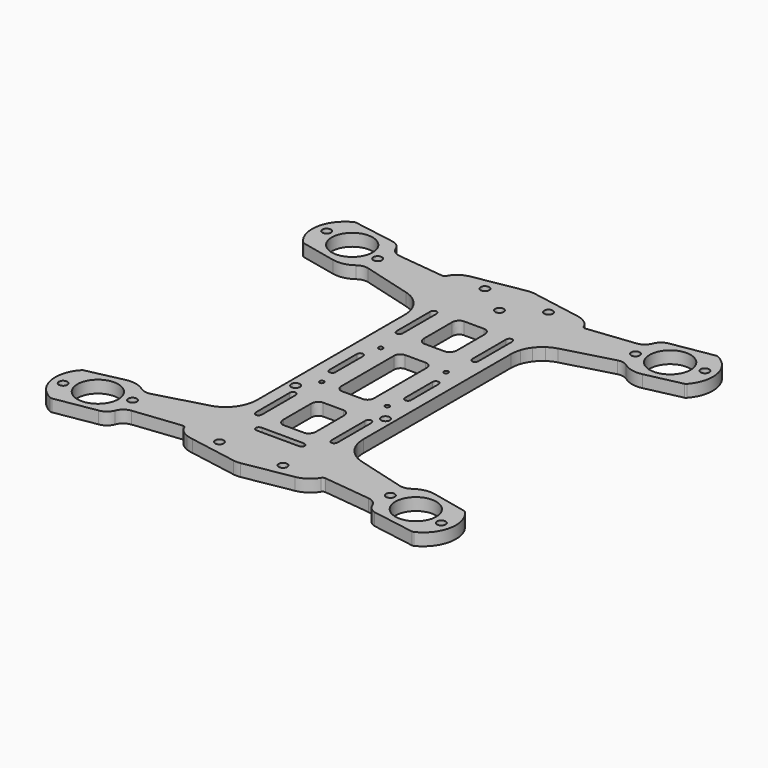
from build123d import *

# Parameters (mm, degrees)
F0_R     = 1.05
F0_R_2   = 5
F0_R_3   = 0.55
F1_DEPTH = 3


# Not quite as in the source:
# - ends of sketch curves that miss each other by under 0.0002 mm in the source are joined


with BuildPart() as f1:
    # F0 (on Top) → F1 (new body)
    with BuildSketch(Plane.XY):
        with BuildLine():
            Line((12.547114, 42.881202), (0.85655, 44.92619))
            ThreePointArc((0.85655, 44.92619), (-0.005, 45.000977), (-0.8665501465, 44.9261908375))
            Line((-0.8665501465, 44.9261908375), (-12.557114, 42.881202))
            ThreePointArc((-12.557114, 42.881202), (-13.3811659144, 42.726197173), (-14.1806832522, 42.4734916576))
            ThreePointArc((-14.1806832522, 42.4734916576), (-14.8442493228, 42.1649785483), (-15.4590972968, 41.7681633969))
            ThreePointArc((-15.4590972968, 41.7681633969), (-15.9947726207, 41.2927995203), (-16.4437235489, 40.7348013706))
            ThreePointArc((-16.4437235489, 40.7348013706), (-16.6010065857, 40.474068763), (-16.7309251323, 40.1986770543))
            ThreePointArc((-16.7309251323, 40.1986770543), (-17.0633376993, 39.8142902587), (-17.5602140107, 39.7076819051))
            Line((-17.5602140107, 39.7076819051), (-28.976888, 40.990102))
            ThreePointArc((-28.976888, 40.990102), (-30.4889144129, 41.6072597908), (-31.4536189137, 42.9250050321))
            ThreePointArc((-31.4536189137, 42.9250050321), (-32.2669695523, 44.1162796633), (-33.5422899426, 44.790247231))
            Line((-33.5422899426, 44.790247231), (-44.024355, 46.547073))
            ThreePointArc((-44.024355, 46.547073), (-44.2703960354, 46.5499421734), (-44.5056712286, 46.4779004714))
            ThreePointArc((-44.5056712286, 46.4779004714), (-48.8678182924, 40.8066015152), (-46.9486082896, 33.9139537381))
            ThreePointArc((-46.9486082896, 33.9139537381), (-46.756758402, 33.7585868692), (-46.5266729937, 33.6691110288))
            Line((-46.5266729937, 33.6691110288), (-37.857414, 31.767143))
            ThreePointArc((-37.857414, 31.767143), (-35.3359003634, 31.7563904573), (-33.0326374155, 32.7826095689))
            ThreePointArc((-33.0326374155, 32.7826095689), (-31.8035160934, 33.3109660693), (-30.4669251472, 33.2524484654))
            Line((-30.4669251472, 33.2524484654), (-18.56562, 29.976315))
            ThreePointArc((-18.56562, 29.976315), (-17.4138061916, 29.5556879599), (-16.3477285533, 28.9498161915))
            ThreePointArc((-16.3477285533, 28.9498161915), (-15.3811482934, 28.1647172936), (-14.555782994, 27.2322850045))
            ThreePointArc((-14.555782994, 27.2322850045), (-13.8911084628, 26.1763608601), (-13.404806368, 25.0273272092))
            ThreePointArc((-13.404806368, 25.0273272092), (-13.1055926689, 23.8032308073), (-13.005, 22.547117))
            Line((-13.005, 22.547117), (-13.005, -22.545163))
            ThreePointArc((-13.005, -22.545163), (-13.1056391598, -23.8016289395), (-13.4049904879, -25.0260568385))
            ThreePointArc((-13.4049904879, -25.0260568385), (-13.8915403308, -26.1754629051), (-14.5565378338, -27.2317031244))
            ThreePointArc((-14.5565378338, -27.2317031244), (-15.3822911127, -28.1644003108), (-16.3492958707, -28.949699189))
            ThreePointArc((-16.3492958707, -28.949699189), (-17.4159327082, -29.5557766888), (-18.5683238155, -29.976536675))
            Line((-18.5683238155, -29.976536675), (-30.468827, -33.252449))
            ThreePointArc((-30.468827, -33.252449), (-31.8054180934, -33.3109660693), (-33.0345392685, -32.7826093676))
            ThreePointArc((-33.0345392685, -32.7826093676), (-35.3378023634, -31.7563904573), (-37.8593158453, -31.7671437053))
            Line((-37.8593158453, -31.7671437053), (-46.528575, -33.669111))
            ThreePointArc((-46.528575, -33.669111), (-46.758660402, -33.7585868692), (-46.9505100734, -33.9139539336))
            ThreePointArc((-46.9505100734, -33.9139539336), (-48.8697202924, -40.8066015152), (-44.5075733347, -46.4779006903))
            ThreePointArc((-44.5075733347, -46.4779006903), (-44.2722980354, -46.5499421734), (-44.0262569999, -46.5470730008))
            Line((-44.0262569999, -46.5470730008), (-34.00125, -44.866851))
            ThreePointArc((-34.00125, -44.866851), (-32.4476725244, -44.2639383706), (-31.4555210863, -42.9250049679))
            ThreePointArc((-31.4555210863, -42.9250049679), (-30.4908164129, -41.6072597908), (-28.9787899602, -40.9901023543))
            Line((-28.9787899602, -40.9901023543), (-17.559317, -39.707367))
            ThreePointArc((-17.559317, -39.707367), (-17.0624979522, -39.8139429564), (-16.7300789977, -40.1982409991))
            ThreePointArc((-16.7300789977, -40.1982409991), (-16.6002219721, -40.4733867622), (-16.4430270568, -40.7338820384))
            ThreePointArc((-16.4430270568, -40.7338820384), (-15.9941324256, -41.2916401808), (-15.4585510869, -41.7667751162))
            ThreePointArc((-15.4585510869, -41.7667751162), (-14.8438267074, -42.1633861463), (-14.1804188227, -42.4717305375))
            ThreePointArc((-14.1804188227, -42.4717305375), (-13.3810245241, -42.7243184881), (-12.557113935, -42.8792484861))
            Line((-12.557113935, -42.8792484861), (-0.86655, -44.924237))
            ThreePointArc((-0.86655, -44.924237), (-0.005, -44.999023), (0.8565499768, -44.9242368672))
            Line((0.8565499768, -44.9242368672), (12.547114, -42.879249))
            ThreePointArc((12.547114, -42.879249), (14.9016711671, -41.9206209342), (16.6479221608, -40.0730510972))
            ThreePointArc((16.6479221608, -40.0730510972), (16.9791102944, -39.7692325356), (17.4218459122, -39.6919257817))
            Line((17.4218459122, -39.6919257817), (28.97879, -40.990102))
            ThreePointArc((28.97879, -40.990102), (30.4908164129, -41.6072597908), (31.4555209137, -42.9250050321))
            ThreePointArc((31.4555209137, -42.9250050321), (32.2688715523, -44.1162796633), (33.5441919426, -44.790247231))
            Line((33.5441919426, -44.790247231), (44.026257, -46.547073))
            ThreePointArc((44.026257, -46.547073), (44.2722980354, -46.5499421734), (44.5075732286, -46.4779004714))
            ThreePointArc((44.5075732286, -46.4779004714), (48.8697202924, -40.8066015152), (46.9505102896, -33.9139537381))
            ThreePointArc((46.9505102896, -33.9139537381), (46.758660402, -33.7585868692), (46.5285749937, -33.6691110288))
            Line((46.5285749937, -33.6691110288), (37.859316, -31.767143))
            ThreePointArc((37.859316, -31.767143), (35.3378023634, -31.7563904573), (33.0345394155, -32.7826095689))
            ThreePointArc((33.0345394155, -32.7826095689), (31.8054180934, -33.3109660693), (30.4688271472, -33.2524484654))
            Line((30.4688271472, -33.2524484654), (18.559028, -29.973977))
            ThreePointArc((18.559028, -29.973977), (17.4064503868, -29.5533376341), (16.3395788739, -28.9474021844))
            ThreePointArc((16.3395788739, -28.9474021844), (15.3725598378, -28.1624472168), (14.5467336983, -27.2300892259))
            ThreePointArc((14.5467336983, -27.2300892259), (13.8816539165, -26.1741955031), (13.3950152055, -25.0250979319))
            ThreePointArc((13.3950152055, -25.0250979319), (13.0956458116, -23.8011576138), (12.995, -22.545163))
            Line((12.995, -22.545163), (12.995, 22.547117))
            ThreePointArc((12.995, 22.547117), (13.0955831803, 23.8028717729), (13.3947679478, 25.0266060173))
            ThreePointArc((13.3947679478, 25.0266060173), (13.8810491707, 26.1753648065), (14.5456781251, 27.2310089064))
            ThreePointArc((14.5456781251, 27.2310089064), (15.3709730893, 28.1631793406), (16.3374399089, 28.9480331332))
            ThreePointArc((16.3374399089, 28.9480331332), (17.4034883055, 29.5537691736), (18.5552417544, 29.9742918988))
            Line((18.5552417544, 29.9742918988), (30.463818, 33.252426))
            ThreePointArc((30.463818, 33.252426), (31.800408437, 33.3109440064), (33.0295292685, 32.7825873676))
            ThreePointArc((33.0295292685, 32.7825873676), (35.3327921796, 31.756367496), (37.8543060546, 31.7671207512))
            Line((37.8543060546, 31.7671207512), (46.523565, 33.669089))
            ThreePointArc((46.523565, 33.669089), (46.7536509796, 33.7585646241), (46.9455010734, 33.9139319336))
            ThreePointArc((46.9455010734, 33.9139319336), (48.8647103142, 40.8065794027), (44.5025641443, 46.4778782976))
            ThreePointArc((44.5025641443, 46.4778782976), (44.2672890354, 46.5499201734), (44.0212479999, 46.5470510008))
            Line((44.0212479999, 46.5470510008), (33.99624, 44.866829))
            ThreePointArc((33.99624, 44.866829), (32.4426631637, 44.2639150954), (31.4505120863, 42.9249819679))
            ThreePointArc((31.4505120863, 42.9249819679), (30.4858074569, 41.6072368251), (28.9737810711, 40.9900793668))
            Line((28.9737810711, 40.9900793668), (17.550624, 39.706931))
            ThreePointArc((17.550624, 39.706931), (17.0537216639, 39.8135552662), (16.7213123855, 40.1979831583))
            ThreePointArc((16.7213123855, 40.1979831583), (16.5913653828, 40.4734865873), (16.434041461, 40.7343266362))
            ThreePointArc((16.434041461, 40.7343266362), (15.9850652254, 41.2924356233), (15.4493465609, 41.76790475))
            ThreePointArc((15.4493465609, 41.76790475), (14.8344418499, 42.164812335), (14.1708039539, 42.4734028797))
            ThreePointArc((14.1708039539, 42.4734028797), (13.371230664, 42.7261632475), (12.547114, 42.881202))
        make_face()
        with Locations((-46.26, -40.3)):
            Circle(F0_R, mode=Mode.SUBTRACT)
        with Locations((-38.895613, -38.887486)):
            Circle(F0_R_2, mode=Mode.SUBTRACT)
        with Locations((-31.53, -37.48)):
            Circle(F0_R, mode=Mode.SUBTRACT)
        with Locations((-7.783131, -40.597392)):
            Circle(F0_R, mode=Mode.SUBTRACT)
        with BuildLine():
            add(Edge.make_bspline(
                [(5.0933147946, -32.4777851358), (5.9933122632, -32.4797918895), (5.9949847622, -31.7297939995), (5.9966572612, -30.9797961094), (5.0966597937, -30.9777888655)],
                knots=[4.7123893072, 4.7123893072, 4.7123893072, 6.2831853072, 6.2831853072, 7.8539813072, 7.8539813072, 7.8539813072], degree=2, weights=[1, 0.7071068967, 1, 0.7071068967, 1]))
            Line((5.0933147946, -32.4777851358), (-5.10666, -32.455041))
            add(Edge.make_bspline(
                [(-5.1033142063, -30.9550448655), (-6.0033121239, -30.9530376206), (-6.0049847619, -31.7030358853), (-6.0066574, -32.4530341501), (-5.10666, -32.455041)],
                knots=[1.570796, 1.570796, 1.570796, 3.1415925, 3.1415925, 4.712389, 4.712389, 4.712389], degree=2, weights=[1, 0.7071067199, 1, 0.7071067199, 1]))
            Line((-5.1033142063, -30.9550448655), (5.0966597937, -30.9777888655))
        make_face(mode=Mode.SUBTRACT)
        with BuildLine():
            add(Edge.make_bspline(
                [(-8.505, -16.4296902941), (-8.5049997549, -15.5296901382), (-9.2549998848, -15.52969), (-10.0050000147, -15.5296898618), (-10.005, -16.4296900177)],
                knots=[1.570796, 1.570796, 1.570796, 3.1415925, 3.1415925, 4.712389, 4.712389, 4.712389], degree=2, weights=[1, 0.7071067199, 1, 0.7071067199, 1]))
            Line((-8.505, -16.4296902941), (-8.505, -26.62969))
            add(Edge.make_bspline(
                [(-10.005, -26.6296900177), (-10.0049999853, -27.5296901735), (-9.2549998554, -27.52969), (-8.5049997255, -27.5296898265), (-8.505, -26.62969)],
                knots=[4.712389, 4.712389, 4.712389, 6.2831855, 6.2831855, 7.853982, 7.853982, 7.853982], degree=2, weights=[1, 0.7071067199, 1, 0.7071067199, 1]))
            Line((-10.005, -26.6296900177), (-10.005, -16.4296900177))
        make_face(mode=Mode.SUBTRACT)
        with BuildLine():
            add(Edge.make_bspline(
                [(-2.5050005196, -15.52969), (-4.0050000294, -15.5296906235), (-4.005, -17.3296900353)],
                knots=[3.141593, 3.141593, 3.141593, 4.712389, 4.712389, 4.712389], degree=2, weights=[1, 0.7071068967, 1]))
            Line((-2.5050005196, -15.52969), (2.495, -15.52969))
            add(Edge.make_bspline(
                [(3.995, -17.3296905882), (3.9950004902, -15.5296893765), (2.495, -15.52969)],
                knots=[1.570796, 1.570796, 1.570796, 3.141593, 3.141593, 3.141593], degree=2, weights=[1, 0.7071065432, 1]))
            Line((3.995, -17.3296905882), (3.995, -25.72969))
            add(Edge.make_bspline(
                [(2.495, -27.52969), (3.9949995098, -27.52969), (3.995, -25.72969)],
                knots=[0, 0, 0, 1.570796, 1.570796, 1.570796], degree=2, weights=[1, 0.7071068967, 1]))
            Line((2.495, -27.52969), (-2.505, -27.52969))
            add(Edge.make_bspline(
                [(-4.005, -25.7296900353), (-4.0049999706, -27.5296894471), (-2.505, -27.52969)],
                knots=[4.712389, 4.712389, 4.712389, 6.283185, 6.283185, 6.283185], degree=2, weights=[1, 0.7071068967, 1]))
            Line((-4.005, -25.7296900353), (-4.005, -17.3296900353))
        make_face(mode=Mode.SUBTRACT)
        with Locations((-11.005, -13.297823)):
            Circle(F0_R, mode=Mode.SUBTRACT)
        with Locations((-8.005, -8.999023)):
            Circle(F0_R_3, mode=Mode.SUBTRACT)
        with Locations((7.773131, -40.597392)):
            Circle(F0_R, mode=Mode.SUBTRACT)
        with Locations((31.53, -37.48)):
            Circle(F0_R, mode=Mode.SUBTRACT)
        with Locations((38.895613, -38.887486)):
            Circle(F0_R_2, mode=Mode.SUBTRACT)
        with Locations((46.26, -40.3)):
            Circle(F0_R, mode=Mode.SUBTRACT)
        with BuildLine():
            add(Edge.make_bspline(
                [(9.995, -16.4296902941), (9.9950002451, -15.5296901382), (9.2450001152, -15.52969), (8.4949999853, -15.5296898618), (8.495, -16.4296900177)],
                knots=[1.570796, 1.570796, 1.570796, 3.1415925, 3.1415925, 4.712389, 4.712389, 4.712389], degree=2, weights=[1, 0.7071067199, 1, 0.7071067199, 1]))
            Line((9.995, -16.4296902941), (9.995, -26.62969))
            add(Edge.make_bspline(
                [(8.495, -26.6296900177), (8.4950000147, -27.5296901735), (9.2450001446, -27.52969), (9.9950002745, -27.5296898265), (9.995, -26.62969)],
                knots=[4.712389, 4.712389, 4.712389, 6.2831855, 6.2831855, 7.853982, 7.853982, 7.853982], degree=2, weights=[1, 0.7071067199, 1, 0.7071067199, 1]))
            Line((8.495, -26.6296900177), (8.495, -16.4296900177))
        make_face(mode=Mode.SUBTRACT)
        with Locations((10.995, -13.297823)):
            Circle(F0_R, mode=Mode.SUBTRACT)
        with Locations((7.995, -8.999023)):
            Circle(F0_R_3, mode=Mode.SUBTRACT)
        with BuildLine():
            ThreePointArc((-8.505, -4.249023), (-9.255, -4.999023), (-10.005, -4.249023))
            Line((-10.005, -4.249023), (-10.005, 4.250977))
            ThreePointArc((-10.005, 4.250977), (-9.255, 5.000977), (-8.505, 4.250977))
            Line((-8.505, 4.250977), (-8.505, -4.249023))
        make_face(mode=Mode.SUBTRACT)
        with BuildLine():
            ThreePointArc((-4.005, 8.125977), (-3.5656601718, 9.1866371718), (-2.505, 9.625977))
            Line((-2.505, 9.625977), (2.495, 9.625977))
            ThreePointArc((2.495, 9.625977), (3.5556601718, 9.1866371718), (3.995, 8.125977))
            Line((3.995, 8.125977), (3.995, -8.124023))
            ThreePointArc((3.995, -8.124023), (3.5556601718, -9.1846831718), (2.495, -9.624023))
            Line((2.495, -9.624023), (-2.505, -9.624023))
            ThreePointArc((-2.505, -9.624023), (-3.5656601718, -9.1846831718), (-4.005, -8.124023))
            Line((-4.005, -8.124023), (-4.005, 8.125977))
        make_face(mode=Mode.SUBTRACT)
        with Locations((-8.005, 9.000977)):
            Circle(F0_R_3, mode=Mode.SUBTRACT)
        with BuildLine():
            add(Edge.make_bspline(
                [(-10.005, 16.4316429823), (-10.0049999853, 15.5316428265), (-9.2549998554, 15.531643), (-8.5049997255, 15.5316431735), (-8.505, 16.4316433294)],
                knots=[4.712389, 4.712389, 4.712389, 6.2831855, 6.2831855, 7.853982, 7.853982, 7.853982], degree=2, weights=[1, 0.7071067199, 1, 0.7071067199, 1]))
            Line((-10.005, 16.4316429823), (-10.005, 26.631643))
            add(Edge.make_bspline(
                [(-8.505, 26.6316427059), (-8.5049997549, 27.5316428618), (-9.2549998848, 27.531643), (-10.0050000147, 27.5316431382), (-10.005, 26.631643)],
                knots=[1.570796, 1.570796, 1.570796, 3.1415925, 3.1415925, 4.712389, 4.712389, 4.712389], degree=2, weights=[1, 0.7071067199, 1, 0.7071067199, 1]))
            Line((-8.505, 26.6316427059), (-8.505, 16.4316433294))
        make_face(mode=Mode.SUBTRACT)
        with BuildLine():
            add(Edge.make_bspline(
                [(-4.005, 17.3316429647), (-4.0049999706, 15.5316435529), (-2.5050004608, 15.531643)],
                knots=[4.712389, 4.712389, 4.712389, 6.283185, 6.283185, 6.283185], degree=2, weights=[1, 0.7071068967, 1]))
            Line((-4.005, 17.3316429647), (-4.005, 25.731643))
            add(Edge.make_bspline(
                [(-2.5050005196, 27.531643), (-4.0050000294, 27.5316423765), (-4.005, 25.731643)],
                knots=[3.141593, 3.141593, 3.141593, 4.712389, 4.712389, 4.712389], degree=2, weights=[1, 0.7071068967, 1]))
            Line((-2.5050005196, 27.531643), (2.495, 27.531643))
            add(Edge.make_bspline(
                [(3.995, 25.7316424118), (3.9950004902, 27.5316436235), (2.495, 27.531643)],
                knots=[1.570796, 1.570796, 1.570796, 3.141593, 3.141593, 3.141593], degree=2, weights=[1, 0.7071065432, 1]))
            Line((3.995, 25.7316424118), (3.995, 17.331643))
            add(Edge.make_bspline(
                [(2.495, 15.531643), (3.9949995098, 15.531643), (3.995, 17.331643)],
                knots=[0, 0, 0, 1.570796, 1.570796, 1.570796], degree=2, weights=[1, 0.7071068967, 1]))
            Line((2.495, 15.531643), (-2.5050004608, 15.531643))
        make_face(mode=Mode.SUBTRACT)
        with Locations((-46.26206, 40.302271)):
            Circle(F0_R, mode=Mode.SUBTRACT)
        with Locations((-38.895873, 38.89185)):
            Circle(F0_R_2, mode=Mode.SUBTRACT)
        with Locations((-31.529686, 37.481428)):
            Circle(F0_R, mode=Mode.SUBTRACT)
        with Locations((-7.783131, 40.599345)):
            Circle(F0_R, mode=Mode.SUBTRACT)
        with Locations((-0.004951, 35.300977)):
            Circle(F0_R, mode=Mode.SUBTRACT)
        with BuildLine():
            ThreePointArc((9.995, -4.249023), (9.245, -4.999023), (8.495, -4.249023))
            Line((8.495, -4.249023), (8.495, 4.250977))
            ThreePointArc((8.495, 4.250977), (9.245, 5.000977), (9.995, 4.250977))
            Line((9.995, 4.250977), (9.995, -4.249023))
        make_face(mode=Mode.SUBTRACT)
        with Locations((7.995, 9.000977)):
            Circle(F0_R_3, mode=Mode.SUBTRACT)
        with BuildLine():
            add(Edge.make_bspline(
                [(8.495, 16.4316429823), (8.4950000147, 15.5316428265), (9.2450001446, 15.531643), (9.9950002745, 15.5316431735), (9.995, 16.4316433294)],
                knots=[4.712389, 4.712389, 4.712389, 6.2831855, 6.2831855, 7.853982, 7.853982, 7.853982], degree=2, weights=[1, 0.7071067199, 1, 0.7071067199, 1]))
            Line((8.495, 16.4316429823), (8.495, 26.631643))
            add(Edge.make_bspline(
                [(9.995, 26.6316427059), (9.9950002451, 27.5316428618), (9.2450001152, 27.531643), (8.4949999853, 27.5316431382), (8.495, 26.631643)],
                knots=[1.570796, 1.570796, 1.570796, 3.1415925, 3.1415925, 4.712389, 4.712389, 4.712389], degree=2, weights=[1, 0.7071067199, 1, 0.7071067199, 1]))
            Line((9.995, 26.6316427059), (9.995, 16.4316433294))
        make_face(mode=Mode.SUBTRACT)
        with Locations((7.773131, 40.599345)):
            Circle(F0_R, mode=Mode.SUBTRACT)
        with Locations((31.53, 37.481428)):
            Circle(F0_R, mode=Mode.SUBTRACT)
        with Locations((38.885873, 38.89185)):
            Circle(F0_R_2, mode=Mode.SUBTRACT)
        with Locations((46.26, 40.302271)):
            Circle(F0_R, mode=Mode.SUBTRACT)
    extrude(amount=F1_DEPTH)


solid = f1.part
